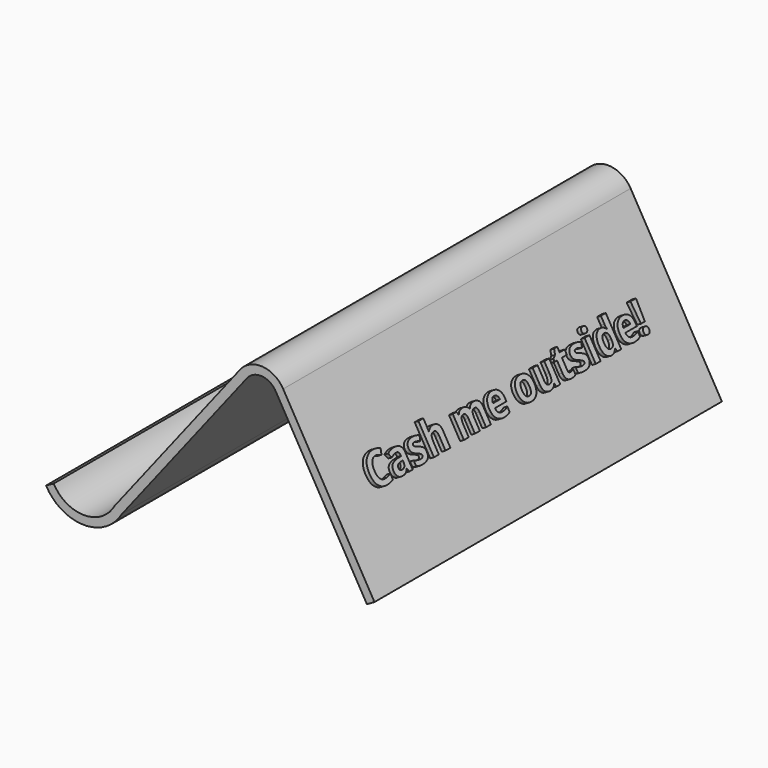
from build123d import *

# Parameters (mm, degrees)
F1_DEPTH     = 100
F2_TEXT_SIZE = 9.3931166067
F3_DEPTH     = 1


# Not quite as in the source:
# - Text() gives the source's letters only with a copy of the font that has no kerning and outlines rounded to 1/6400 em; it was checked with that copy


with BuildPart() as f1:
    # F0 (on Front) → F1 (new body)
    with BuildSketch(Plane.XZ):
        with BuildLine():
            ThreePointArc((4.4516113795, 36.3623516559), (-0.3275242067, 39.345298856), (-5.4729582171, 37.0512587965))
            Line((-5.4729582171, 37.0512587965), (-34.3901541668, 0))
            ThreePointArc((-34.3901541668, 0), (-41.3901541668, -4.1270166538), (-48.3901541668, 0))
            Line((-48.3901541668, 0), (-50.1401541668, -0.9682458366))
            ThreePointArc((-50.1401541668, -0.9682458366), (-41.4733605117, -6.126670483), (-32.7219271517, -1.1131815543))
            Line((-32.7219271517, -1.1131815543), (-3.8963089066, 35.8207398199))
            ThreePointArc((-3.8963089066, 35.8207398199), (-0.4660195663, 37.3500998596), (2.7200708245, 35.3614683928))
            Line((2.7200708245, 35.3614683928), (23.7386193484, -1.000883263))
            Line((23.7386193484, -1.000883263), (25.4701599035, 0))
            Line((25.4701599035, 0), (4.4516113795, 36.3623516559))
        make_face()
    extrude(amount=F1_DEPTH)

    # F2 (on face) → F3 (join)
    with BuildSketch(Plane(origin=(19.0913665344, 0, 11.0353922565), x_dir=(0, 1, 0), z_dir=(0.8657702775, 0, 0.5004416315))):
        with Locations((-90, 4.8721496443)):
            Text('Cash me outside!', F2_TEXT_SIZE, font='Open Sans', font_style=FontStyle.BOLD, text_align=(TextAlign.LEFT, TextAlign.BOTTOM))
    extrude(amount=F3_DEPTH)


solid = f1.part
